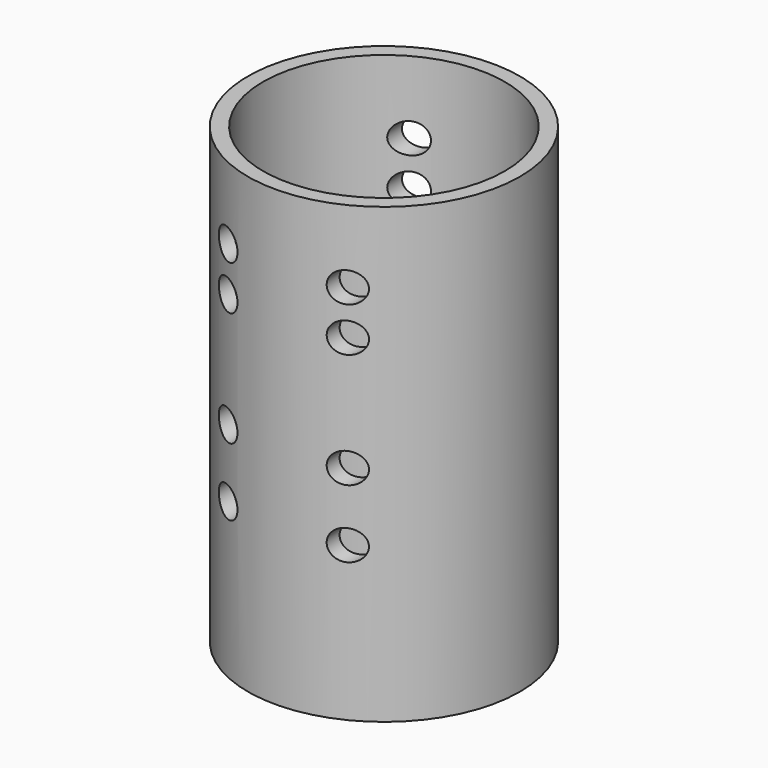
from build123d import *

# Parameters (mm, degrees)
F0_R          = 57.15
F0_R_2        = 50.8
F1_DEPTH      = 190.5
F2_R          = 6.35
F3_DEPTH      = 76.2
F3_DEPTH_BACK = 76.2


# Not quite as in the source:
# - a feature names something its author has since deleted; it is built from what else it names


with BuildPart() as f1:
    # F0 (on Top) → F1 (new body)
    with BuildSketch(Plane.XY):
        Circle(F0_R)
        Circle(F0_R_2, mode=Mode.SUBTRACT)
    extrude(amount=F1_DEPTH)

    # F2 (on Front) → F3 (cut, two sides)
    with BuildSketch(Plane.XZ) as f3_sk:
        with Locations((25.4, 93.2306411874)):
            Circle(F2_R)
        with Locations((25.3999390757, 160.0650958556)):
            Circle(F2_R)
        with Locations((25.4053702194, 141.4302072382)):
            Circle(F2_R)
        with Locations((25.3971906698, 64.7056564309)):
            Circle(F2_R)
        with Locations((-24.5366245508, 93.2306411874)):
            Circle(F2_R)
        with Locations((-24.5312543315, 141.4302072382)):
            Circle(F2_R)
        with Locations((-24.5366245508, 160.0650958556)):
            Circle(F2_R)
        with Locations((-24.536624004, 64.77)):
            Circle(F2_R)
    extrude(amount=-F3_DEPTH, mode=Mode.SUBTRACT)
    extrude(f3_sk.sketch, amount=F3_DEPTH_BACK, mode=Mode.SUBTRACT)


solid = f1.part
